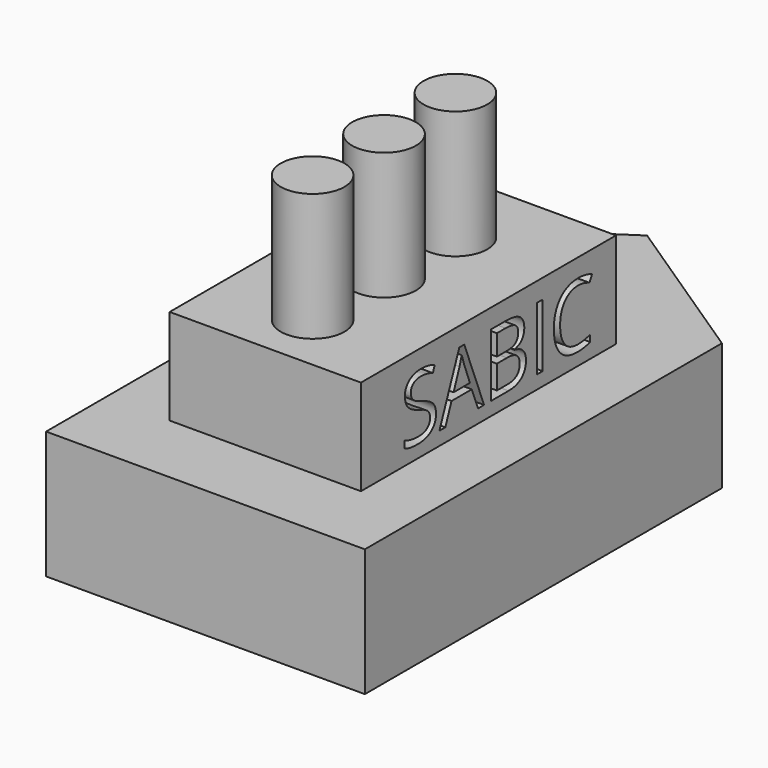
from build123d import *

# Parameters (mm, degrees)
F1_DEPTH     = 25.4
F2_W         = 38.1
F2_H         = 63.5
F3_DEPTH     = 19.05
F4_R         = 6.35
F5_DEPTH     = 25.4
F6_TEXT_SIZE = 17.5881251279
F7_DEPTH     = 40.132


# Not quite as in the source:
# - Text() gives the source's letters only with a copy of the font that has no kerning and outlines rounded to 1/6400 em; it was checked with that copy


with BuildPart() as f1:
    # F0 (on Top) → F1 (new body)
    with BuildSketch(Plane.XY):
        Polygon((0, 59.7160486747), (-31.75, 38.6554812559), (-31.75, -50.2445187441), (31.75, -50.2445187441), (31.75, 38.6554812559), align=None)
    extrude(amount=F1_DEPTH)

    # F2 (on face) → F3 (join)
    with BuildSketch(Plane.XY.offset(25.4)):
        with Locations((0, -3.5975724459)):
            Rectangle(F2_W, F2_H)
    extrude(amount=F3_DEPTH)

    # F4 (on face) → F5 (join)
    with BuildSketch(Plane.XY.offset(44.45)):
        with Locations((0, 11.9895519281)):
            Circle(F4_R)
        with Locations((0, -5.7904480719)):
            Circle(F4_R)
        with Locations((0, -23.5704480719)):
            Circle(F4_R)
    extrude(amount=F5_DEPTH)

    # F6 (on face) → F7 (cut)
    with BuildSketch(Plane.YZ.offset(19.05)):
        with Locations((-25.470810011, 28.0610620975)):
            Text('SABIC', F6_TEXT_SIZE, font='Open Sans', text_align=(TextAlign.LEFT, TextAlign.BOTTOM))
    extrude(amount=-F7_DEPTH, mode=Mode.SUBTRACT)


solid = f1.part
